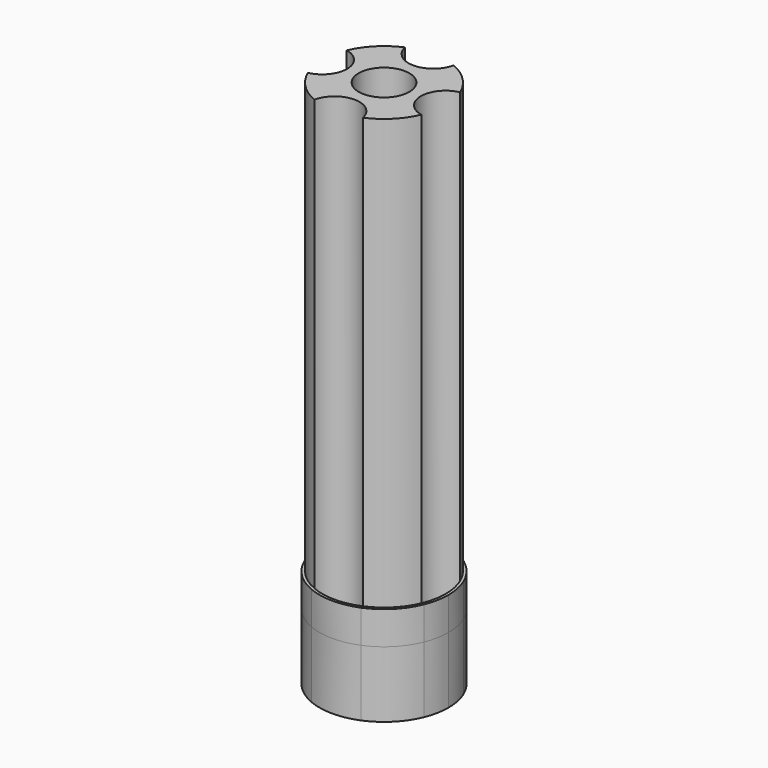
from build123d import *

# Parameters (mm, degrees)
F1_DEPTH = 5.08
F0_R     = 1.9431
F2_DEPTH = 35.56
F3_DEPTH = 2.54


with BuildPart() as f1:
    # F0 (on Top) → F1 (new body)
    with BuildSketch(Plane.XY):
        with BuildLine():
            ThreePointArc((4.5748770777, -1.8980802732), (4.8575495451, -0.9676886984), (4.953, 0))
            ThreePointArc((4.953, 0), (4.8575495451, 0.9676886984), (4.5748770777, 1.8980802732))
            ThreePointArc((4.5748770777, 1.8980802732), (4.4639983721, 1.8853223864), (4.3540571046, 1.8660930149))
            ThreePointArc((4.3540571046, 1.8660930149), (4.640351297, 0.9525), (4.7371, 0))
            ThreePointArc((4.7371, 0), (4.640351297, -0.9525), (4.3540571046, -1.8660930149))
            ThreePointArc((4.3540571046, -1.8660930149), (4.4639983721, -1.8853223864), (4.5748770777, -1.8980802732))
        make_face()
        with BuildLine():
            ThreePointArc((4.3540571046, 1.8660930149), (4.4639983721, 1.8853223864), (4.5748770777, 1.8980802732))
            ThreePointArc((4.5748770777, 1.8980802732), (3.5022998872, 3.5022998872), (1.8980802732, 4.5748770777))
            ThreePointArc((1.8980802732, 4.5748770777), (1.8853223864, 4.4639983721), (1.8660930149, 4.3540571046))
            ThreePointArc((1.8660930149, 4.3540571046), (3.3496355332, 3.3496355332), (4.3540571046, 1.8660930149))
        make_face()
        with BuildLine():
            ThreePointArc((1.8980802732, -4.5748770777), (3.5022998872, -3.5022998872), (4.5748770777, -1.8980802732))
            ThreePointArc((4.5748770777, -1.8980802732), (4.4639983721, -1.8853223864), (4.3540571046, -1.8660930149))
            ThreePointArc((4.3540571046, -1.8660930149), (3.3496355332, -3.3496355332), (1.8660930149, -4.3540571046))
            ThreePointArc((1.8660930149, -4.3540571046), (1.8853223864, -4.4639983721), (1.8980802732, -4.5748770777))
        make_face()
        with BuildLine():
            ThreePointArc((1.8660930149, 4.3540571046), (1.8853223864, 4.4639983721), (1.8980802732, 4.5748770777))
            ThreePointArc((1.8980802732, 4.5748770777), (0, 4.953), (-1.8980802732, 4.5748770777))
            ThreePointArc((-1.8980802732, 4.5748770777), (-1.8853223864, 4.4639983721), (-1.8660930149, 4.3540571046))
            ThreePointArc((-1.8660930149, 4.3540571046), (0, 4.7371), (1.8660930149, 4.3540571046))
        make_face()
        with BuildLine():
            ThreePointArc((-1.8980802732, -4.5748770777), (0, -4.953), (1.8980802732, -4.5748770777))
            ThreePointArc((1.8980802732, -4.5748770777), (1.8853223864, -4.4639983721), (1.8660930149, -4.3540571046))
            ThreePointArc((1.8660930149, -4.3540571046), (0, -4.7371), (-1.8660930149, -4.3540571046))
            ThreePointArc((-1.8660930149, -4.3540571046), (-1.8853223864, -4.4639983721), (-1.8980802732, -4.5748770777))
        make_face()
        with BuildLine():
            ThreePointArc((-1.8660930149, 4.3540571046), (-1.8853223864, 4.4639983721), (-1.8980802732, 4.5748770777))
            ThreePointArc((-1.8980802732, 4.5748770777), (-3.5022998872, 3.5022998872), (-4.5748770777, 1.8980802732))
            ThreePointArc((-4.5748770777, 1.8980802732), (-4.4639983721, 1.8853223864), (-4.3540571046, 1.8660930149))
            ThreePointArc((-4.3540571046, 1.8660930149), (-3.3496355332, 3.3496355332), (-1.8660930149, 4.3540571046))
        make_face()
        with BuildLine():
            ThreePointArc((-4.5748770777, -1.8980802732), (-3.5022998872, -3.5022998872), (-1.8980802732, -4.5748770777))
            ThreePointArc((-1.8980802732, -4.5748770777), (-1.8853223864, -4.4639983721), (-1.8660930149, -4.3540571046))
            ThreePointArc((-1.8660930149, -4.3540571046), (-3.3496355332, -3.3496355332), (-4.3540571046, -1.8660930149))
            ThreePointArc((-4.3540571046, -1.8660930149), (-4.4639983721, -1.8853223864), (-4.5748770777, -1.8980802732))
        make_face()
        with BuildLine():
            ThreePointArc((-4.3540571046, 1.8660930149), (-4.4639983721, 1.8853223864), (-4.5748770777, 1.8980802732))
            ThreePointArc((-4.5748770777, 1.8980802732), (-4.953, 0), (-4.5748770777, -1.8980802732))
            ThreePointArc((-4.5748770777, -1.8980802732), (-4.4639983721, -1.8853223864), (-4.3540571046, -1.8660930149))
            ThreePointArc((-4.3540571046, -1.8660930149), (-4.7371, 0), (-4.3540571046, 1.8660930149))
        make_face()
    extrude(amount=-F1_DEPTH)


with BuildPart() as f2:
    # F0 (on Top) → F2 (new body)
    with BuildSketch(Plane.XY):
        with BuildLine():
            ThreePointArc((4.3540571046, -1.8660930149), (2.8321, 0), (4.3540571046, 1.8660930149))
            ThreePointArc((4.3540571046, 1.8660930149), (3.3496355332, 3.3496355332), (1.8660930149, 4.3540571046))
            ThreePointArc((1.8660930149, 4.3540571046), (0, 2.8321), (-1.8660930149, 4.3540571046))
            ThreePointArc((-1.8660930149, 4.3540571046), (-3.3496355332, 3.3496355332), (-4.3540571046, 1.8660930149))
            ThreePointArc((-4.3540571046, 1.8660930149), (-2.8321, 0), (-4.3540571046, -1.8660930149))
            ThreePointArc((-4.3540571046, -1.8660930149), (-3.3496355332, -3.3496355332), (-1.8660930149, -4.3540571046))
            ThreePointArc((-1.8660930149, -4.3540571046), (0, -2.8321), (1.8660930149, -4.3540571046))
            ThreePointArc((1.8660930149, -4.3540571046), (3.3496355332, -3.3496355332), (4.3540571046, -1.8660930149))
        make_face()
        Circle(F0_R, mode=Mode.SUBTRACT)
    extrude(amount=F2_DEPTH)


with BuildPart() as f3:
    # F0 (on Top) → F3 (new body)
    with BuildSketch(Plane.XY):
        with BuildLine():
            ThreePointArc((4.5748770777, -1.8980802732), (4.8575495451, -0.9676886984), (4.953, 0))
            ThreePointArc((4.953, 0), (4.8575495451, 0.9676886984), (4.5748770777, 1.8980802732))
            ThreePointArc((4.5748770777, 1.8980802732), (4.4639983721, 1.8853223864), (4.3540571046, 1.8660930149))
            ThreePointArc((4.3540571046, 1.8660930149), (4.640351297, 0.9525), (4.7371, 0))
            ThreePointArc((4.7371, 0), (4.640351297, -0.9525), (4.3540571046, -1.8660930149))
            ThreePointArc((4.3540571046, -1.8660930149), (4.4639983721, -1.8853223864), (4.5748770777, -1.8980802732))
        make_face()
        with BuildLine():
            ThreePointArc((4.3540571046, 1.8660930149), (4.4639983721, 1.8853223864), (4.5748770777, 1.8980802732))
            ThreePointArc((4.5748770777, 1.8980802732), (3.5022998872, 3.5022998872), (1.8980802732, 4.5748770777))
            ThreePointArc((1.8980802732, 4.5748770777), (1.8853223864, 4.4639983721), (1.8660930149, 4.3540571046))
            ThreePointArc((1.8660930149, 4.3540571046), (3.3496355332, 3.3496355332), (4.3540571046, 1.8660930149))
        make_face()
        with BuildLine():
            ThreePointArc((1.8980802732, -4.5748770777), (3.5022998872, -3.5022998872), (4.5748770777, -1.8980802732))
            ThreePointArc((4.5748770777, -1.8980802732), (4.4639983721, -1.8853223864), (4.3540571046, -1.8660930149))
            ThreePointArc((4.3540571046, -1.8660930149), (3.3496355332, -3.3496355332), (1.8660930149, -4.3540571046))
            ThreePointArc((1.8660930149, -4.3540571046), (1.8853223864, -4.4639983721), (1.8980802732, -4.5748770777))
        make_face()
        with BuildLine():
            ThreePointArc((1.8660930149, 4.3540571046), (1.8853223864, 4.4639983721), (1.8980802732, 4.5748770777))
            ThreePointArc((1.8980802732, 4.5748770777), (0, 4.953), (-1.8980802732, 4.5748770777))
            ThreePointArc((-1.8980802732, 4.5748770777), (-1.8853223864, 4.4639983721), (-1.8660930149, 4.3540571046))
            ThreePointArc((-1.8660930149, 4.3540571046), (0, 4.7371), (1.8660930149, 4.3540571046))
        make_face()
        with BuildLine():
            ThreePointArc((-1.8980802732, -4.5748770777), (0, -4.953), (1.8980802732, -4.5748770777))
            ThreePointArc((1.8980802732, -4.5748770777), (1.8853223864, -4.4639983721), (1.8660930149, -4.3540571046))
            ThreePointArc((1.8660930149, -4.3540571046), (0, -4.7371), (-1.8660930149, -4.3540571046))
            ThreePointArc((-1.8660930149, -4.3540571046), (-1.8853223864, -4.4639983721), (-1.8980802732, -4.5748770777))
        make_face()
        with BuildLine():
            ThreePointArc((-1.8660930149, 4.3540571046), (-1.8853223864, 4.4639983721), (-1.8980802732, 4.5748770777))
            ThreePointArc((-1.8980802732, 4.5748770777), (-3.5022998872, 3.5022998872), (-4.5748770777, 1.8980802732))
            ThreePointArc((-4.5748770777, 1.8980802732), (-4.4639983721, 1.8853223864), (-4.3540571046, 1.8660930149))
            ThreePointArc((-4.3540571046, 1.8660930149), (-3.3496355332, 3.3496355332), (-1.8660930149, 4.3540571046))
        make_face()
        with BuildLine():
            ThreePointArc((-4.5748770777, -1.8980802732), (-3.5022998872, -3.5022998872), (-1.8980802732, -4.5748770777))
            ThreePointArc((-1.8980802732, -4.5748770777), (-1.8853223864, -4.4639983721), (-1.8660930149, -4.3540571046))
            ThreePointArc((-1.8660930149, -4.3540571046), (-3.3496355332, -3.3496355332), (-4.3540571046, -1.8660930149))
            ThreePointArc((-4.3540571046, -1.8660930149), (-4.4639983721, -1.8853223864), (-4.5748770777, -1.8980802732))
        make_face()
        with BuildLine():
            ThreePointArc((-4.3540571046, 1.8660930149), (-4.4639983721, 1.8853223864), (-4.5748770777, 1.8980802732))
            ThreePointArc((-4.5748770777, 1.8980802732), (-4.953, 0), (-4.5748770777, -1.8980802732))
            ThreePointArc((-4.5748770777, -1.8980802732), (-4.4639983721, -1.8853223864), (-4.3540571046, -1.8660930149))
            ThreePointArc((-4.3540571046, -1.8660930149), (-4.7371, 0), (-4.3540571046, 1.8660930149))
        make_face()
    extrude(amount=F3_DEPTH)


solid = Compound([f1.part, f2.part, f3.part])
